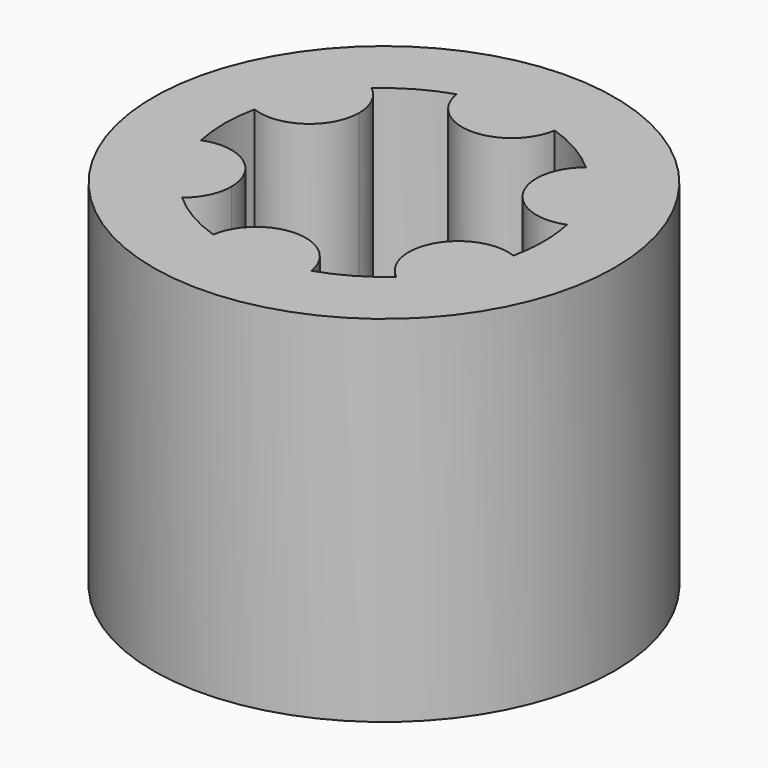
from build123d import *

# Parameters (mm, degrees)
F0_R     = 3.25
F1_DEPTH = 5


with BuildPart() as f1:
    # F0 (on Top) → F1 (new body)
    with BuildSketch(Plane.XY):
        Circle(F0_R)
        with BuildLine():
            ThreePointArc((2.1999961154, 0.4717171738), (2.2374641069, 0.2371800374), (2.25, 0))
            ThreePointArc((2.25, 0), (2.2374641069, -0.2371800374), (2.1999961154, -0.4717171738))
            ThreePointArc((2.1999961154, -0.4717171738), (2.5256218299, -0.7287723318), (2.6485571585, -1.125))
            ThreePointArc((2.6485571585, -1.125), (2.2501959894, -1.7566755621), (1.5085171137, -1.6693939373))
            ThreePointArc((1.5085171137, -1.6693939373), (1.125, -1.9485571585), (0.6914790018, -2.1411111111))
            ThreePointArc((0.6914790018, -2.1411111111), (0.6978664991, -2.1953891093), (0.7, -2.25))
            ThreePointArc((0.7, -2.25), (-0.0546108907, -2.9478664991), (-0.6914790018, -2.1411111111))
            ThreePointArc((-0.6914790018, -2.1411111111), (-1.125, -1.9485571585), (-1.5085171137, -1.6693939373))
            ThreePointArc((-1.5085171137, -1.6693939373), (-2.5547749412, -1.475), (-2.1999961154, -0.4717171738))
            ThreePointArc((-2.1999961154, -0.4717171738), (-2.25, 0), (-2.1999961154, 0.4717171738))
            ThreePointArc((-2.1999961154, 0.4717171738), (-2.5547749412, 1.475), (-1.5085171137, 1.6693939373))
            ThreePointArc((-1.5085171137, 1.6693939373), (-1.125, 1.9485571585), (-0.6914790018, 2.1411111111))
            ThreePointArc((-0.6914790018, 2.1411111111), (-0.0546108907, 2.9478664991), (0.7, 2.25))
            ThreePointArc((0.7, 2.25), (0.6978664991, 2.1953891093), (0.6914790018, 2.1411111111))
            ThreePointArc((0.6914790018, 2.1411111111), (1.125, 1.9485571585), (1.5085171137, 1.6693939373))
            ThreePointArc((1.5085171137, 1.6693939373), (2.2501959894, 1.7566755621), (2.6485571585, 1.125))
            ThreePointArc((2.6485571585, 1.125), (2.5256218299, 0.7287723318), (2.1999961154, 0.4717171738))
        make_face(mode=Mode.SUBTRACT)
        with BuildLine():
            ThreePointArc((1.5085171137, 1.6693939373), (1.9485571585, 1.125), (2.1999961154, 0.4717171738))
            ThreePointArc((2.1999961154, 0.4717171738), (2.5256218299, 0.7287723318), (2.6485571585, 1.125))
            ThreePointArc((2.6485571585, 1.125), (2.2501959894, 1.7566755621), (1.5085171137, 1.6693939373))
        make_face()
        with BuildLine():
            ThreePointArc((2.6485571585, -1.125), (2.5256218299, -0.7287723318), (2.1999961154, -0.4717171738))
            ThreePointArc((2.1999961154, -0.4717171738), (1.9485571585, -1.125), (1.5085171137, -1.6693939373))
            ThreePointArc((1.5085171137, -1.6693939373), (2.2501959894, -1.7566755621), (2.6485571585, -1.125))
        make_face()
        with BuildLine():
            ThreePointArc((-0.6914790018, 2.1411111111), (0, 2.25), (0.6914790018, 2.1411111111))
            ThreePointArc((0.6914790018, 2.1411111111), (0.6978664991, 2.1953891093), (0.7, 2.25))
            ThreePointArc((0.7, 2.25), (-0.0546108907, 2.9478664991), (-0.6914790018, 2.1411111111))
        make_face()
        with BuildLine():
            ThreePointArc((0.7, -2.25), (0.6978664991, -2.1953891093), (0.6914790018, -2.1411111111))
            ThreePointArc((0.6914790018, -2.1411111111), (0, -2.25), (-0.6914790018, -2.1411111111))
            ThreePointArc((-0.6914790018, -2.1411111111), (-0.0546108907, -2.9478664991), (0.7, -2.25))
        make_face()
        with BuildLine():
            ThreePointArc((-2.1999961154, 0.4717171738), (-1.9485571585, 1.125), (-1.5085171137, 1.6693939373))
            ThreePointArc((-1.5085171137, 1.6693939373), (-2.5547749412, 1.475), (-2.1999961154, 0.4717171738))
        make_face()
        with BuildLine():
            ThreePointArc((-2.1999961154, -0.4717171738), (-2.5547749412, -1.475), (-1.5085171137, -1.6693939373))
            ThreePointArc((-1.5085171137, -1.6693939373), (-1.9485571585, -1.125), (-2.1999961154, -0.4717171738))
        make_face()
        with BuildLine():
            ThreePointArc((1.5085171137, 1.6693939373), (1.3423393759, 0.775), (2.1999961154, 0.4717171738))
            ThreePointArc((2.1999961154, 0.4717171738), (1.9485571585, 1.125), (1.5085171137, 1.6693939373))
        make_face()
        with BuildLine():
            ThreePointArc((1.5085171137, -1.6693939373), (1.9485571585, -1.125), (2.1999961154, -0.4717171738))
            ThreePointArc((2.1999961154, -0.4717171738), (1.3423393759, -0.775), (1.5085171137, -1.6693939373))
        make_face()
        with BuildLine():
            ThreePointArc((-0.6914790018, 2.1411111111), (0, 1.55), (0.6914790018, 2.1411111111))
            ThreePointArc((0.6914790018, 2.1411111111), (0, 2.25), (-0.6914790018, 2.1411111111))
        make_face()
        with BuildLine():
            ThreePointArc((-0.6914790018, -2.1411111111), (0, -2.25), (0.6914790018, -2.1411111111))
            ThreePointArc((0.6914790018, -2.1411111111), (0, -1.55), (-0.6914790018, -2.1411111111))
        make_face()
        with BuildLine():
            ThreePointArc((-1.2485571585, 1.125), (-1.3168815965, 1.4266388309), (-1.5085171137, 1.6693939373))
            ThreePointArc((-1.5085171137, 1.6693939373), (-1.9485571585, 1.125), (-2.1999961154, 0.4717171738))
            ThreePointArc((-2.1999961154, 0.4717171738), (-1.5523294903, 0.5479353287), (-1.2485571585, 1.125))
        make_face()
        with BuildLine():
            ThreePointArc((-2.1999961154, -0.4717171738), (-1.9485571585, -1.125), (-1.5085171137, -1.6693939373))
            ThreePointArc((-1.5085171137, -1.6693939373), (-1.3168815965, -1.4266388309), (-1.2485571585, -1.125))
            ThreePointArc((-1.2485571585, -1.125), (-1.5523294903, -0.5479353287), (-2.1999961154, -0.4717171738))
        make_face()
    extrude(amount=F1_DEPTH)


solid = f1.part
